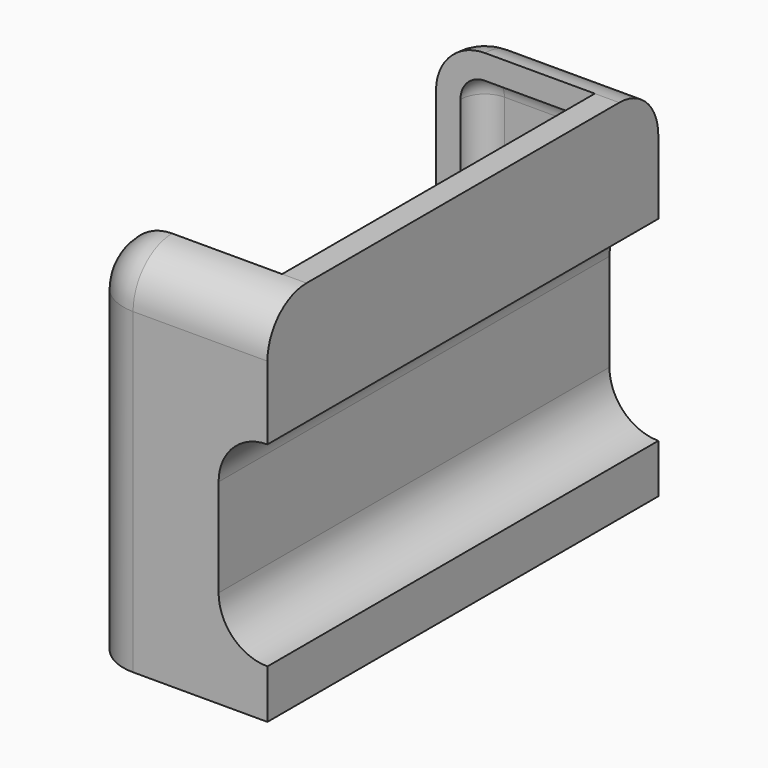
from build123d import *

# Parameters (mm, degrees)
F0_W        = 19.05
F0_H        = 50.8
F1_DEPTH    = 38.1
F2_R        = 5.08
F3_W        = 5.08
F3_H        = 20.32
F4_DEPTH    = 50.8
F5_T        = 2.54
F5_T3_DEPTH = 55.88
F6_R        = 5.07999
F7_R        = 0.635
F8_DEPTH    = 21.59


# Not quite as in the source:
# - a fillet or chamfer is up to 0.001 mm smaller than in the source, because OpenCascade refuses the exact size
# - a shell that OpenCascade refuses in one call is made with other operations: the cavity is built on its own and cut out


with BuildPart() as f1:
    # F0 (on Top) → F1 (new body)
    with BuildSketch(Plane.XY):
        Rectangle(F0_W, F0_H)
    extrude(amount=F1_DEPTH)

    # F2
    f2_edges = [f1.edges().sort_by_distance(p)[0] for p in [
        (0, -25.4, 38.1),
        (0, 25.4, 38.1),
        (-9.525, -25.4, 19.05),
        (-9.525, 0, 38.1),
        (-9.525, 25.4, 19.05),
    ]]
    fillet(f2_edges, radius=F2_R)

    # F3 (on face) → F4 (cut)
    with BuildSketch(Plane.XZ.offset(25.4)):
        with Locations((6.985, 15.24)):
            Rectangle(F3_W, F3_H)
    extrude(amount=-F4_DEPTH, mode=Mode.SUBTRACT)

    # F5: shell of thickness 2.54, made by hand


with BuildPart() as f5_core1:
    # F5_t2: copy of F1
    add(f1.part)

    # the walls: a layer under each face that stays
    f5_faces = [f5_core1.faces().sort_by_distance(p)[0] for p in [
        (2.54, -25.4, 16.51),
        (9.525, 0, 2.54),
        (6.985, 0, 5.08),
        (4.445, 0, 15.24),
        (6.985, 0, 25.4),
        (9.525, 0, 31.75),
        (2.54, -23.9121024484, 36.6121024484),
        (-8.0371024484, -23.9121024484, 16.51),
        (0, 0, 0),
        (2.54, 25.4, 16.51),
        (2.54, 23.9121024484, 36.6121024484),
        (-8.0371024484, -22.86, 35.56),
        (-8.0371024484, 23.9121024484, 16.51),
        (-8.0371024484, 22.86, 35.56),
    ]]
    thicken(f5_faces, amount=-F5_T, mode=Mode.SUBTRACT)

    # F5_s4 → F5_t3 (cut)
    with BuildSketch(Plane.XZ.offset(-27.94)):
        Polygon((4.4704, 5.1054), (4.445, 2.54), (1.905, 2.54), (1.905, 5.08), align=None)
        Polygon((4.4704, 25.3746), (1.905, 25.4), (1.905, 27.94), (4.445, 27.94), align=None)
    extrude(amount=F5_T3_DEPTH, mode=Mode.SUBTRACT)


with BuildPart() as f1_1:
    add(f1.part)

    # what is left inside the walls is the cavity
    f5_cavity = [f5_core1.part.solids().sort_by_distance(p)[0] for p in [
        (-9.4996, 0, 22.86),
    ]]
    add(f5_cavity, mode=Mode.SUBTRACT)

    # F6 (radius 5.08 in the source; OpenCascade refuses exactly that, so slightly less here)
    f6_edges = [f1_1.edges().sort_by_distance(p)[0] for p in [
        (4.445, 0, 5.08),
        (4.445, 0, 25.4),
    ]]
    fillet(f6_edges, radius=F6_R)

    # F7 (on Front) → F8 (cut, symmetric)
    with BuildSketch(Plane.XZ):
        with Locations((6.985, 36.83)):
            Circle(F7_R)
    extrude(amount=F8_DEPTH, both=True, mode=Mode.SUBTRACT)


solid = f1_1.part
